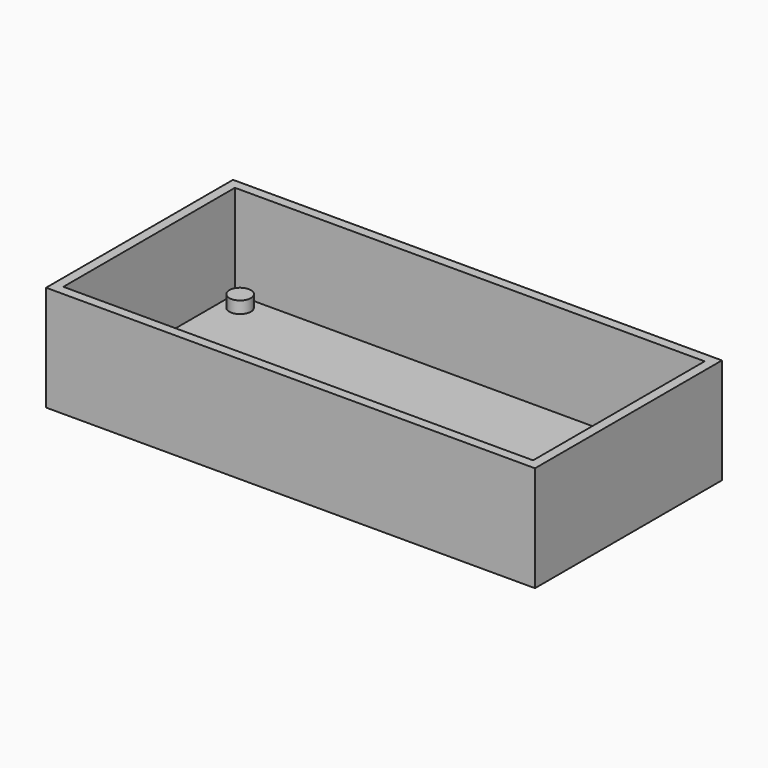
from build123d import *

# Parameters (mm, degrees)
F0_R     = 2.25
F1_DEPTH = 5
F0_W     = 53.1
F0_H     = 44.7
F2_DEPTH = 2.5
F6_DEPTH = 44.8
F7_W     = 101.9
F7_H     = 48.7
F7_W_2   = 97.9
F7_H_2   = 44.7
F8_DEPTH = 22


# Not quite as in the source:
# - a feature names something its author has since deleted; it is built from what else it names
# - the program builds the solid bodies; features that only make, move or delete a surface that nothing else refers to are left out


with BuildPart() as f1:
    # F0 (on Top) → F1 (new body)
    with BuildSketch(Plane.XY):
        with Locations((-22.8803921491, 19.1126316786)):
            Circle(F0_R)
    extrude(amount=F1_DEPTH)


with BuildPart() as f2:
    # F0 (on Top) → F2 (new body)
    with BuildSketch(Plane.XY):
        Rectangle(F0_W, F0_H)
        with Locations((-22.8803921491, 19.1126316786)):
            Circle(F0_R, mode=Mode.SUBTRACT)
    extrude(amount=F2_DEPTH)

    # F6 (add): a face of the model
    f6_faces = [f2.faces().sort_by_distance(p)[0] for p in [
        (26.55, 0, 1.25),
    ]]
    extrude(f6_faces, amount=F6_DEPTH)

    # F7 (on Top) → F8 (join)
    with BuildSketch(Plane.XY):
        with Locations((22.4, 0)):
            Rectangle(F7_W, F7_H)
        with Locations((22.4, 0)):
            Rectangle(F7_W_2, F7_H_2, mode=Mode.SUBTRACT)
    extrude(amount=F8_DEPTH)


solid = Compound([f1.part, f2.part])
